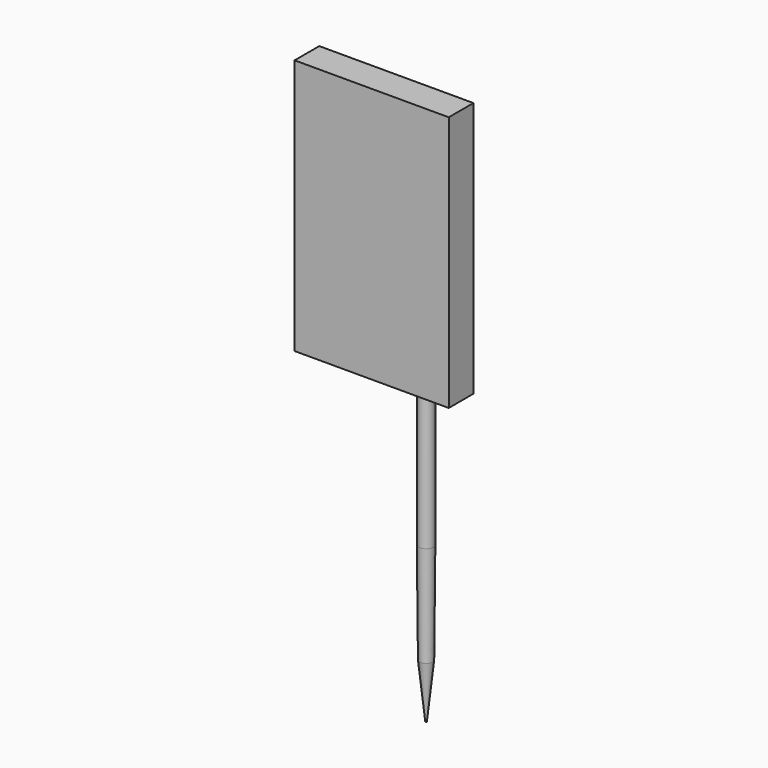
from build123d import *

# Parameters (mm, degrees)
F0_W     = 85
F0_H     = 141.1
F1_DEPTH = 17
F2_R     = 4
F3_DEPTH = 77
F4_R     = 4
F5_DEPTH = 55.9
F5_TAPER = 0.5
F6_R     = 3.5121680905
F7_DEPTH = 30
F7_TAPER = 6


with BuildPart() as f1:
    # F0 (on Front) → F1 (new body)
    with BuildSketch(Plane.XZ):
        with Locations((42.5, 70.55)):
            Rectangle(F0_W, F0_H)
    extrude(amount=F1_DEPTH)

    # F2 (on face) → F3 (join)
    with BuildSketch(Plane(origin=(0, 0, 0), x_dir=(1, 0, 0), z_dir=(0, 0, -1))):
        with Locations((64.5, 7)):
            Circle(F2_R)
    extrude(amount=F3_DEPTH)

    # F4 (on face) → F5 (join)
    with BuildSketch(Plane(origin=(0, 0, -77), x_dir=(1, 0, 0), z_dir=(0, 0, -1))):
        with Locations((64.5, 7)):
            Circle(F4_R)
    extrude(amount=F5_DEPTH, taper=F5_TAPER)

    # F6 (on face) → F7 (join)
    with BuildSketch(Plane(origin=(0, 0, -132.9), x_dir=(1, 0, 0), z_dir=(0, 0, -1))):
        with Locations((64.5, 7)):
            Circle(F6_R)
    extrude(amount=F7_DEPTH, taper=F7_TAPER)


solid = f1.part
